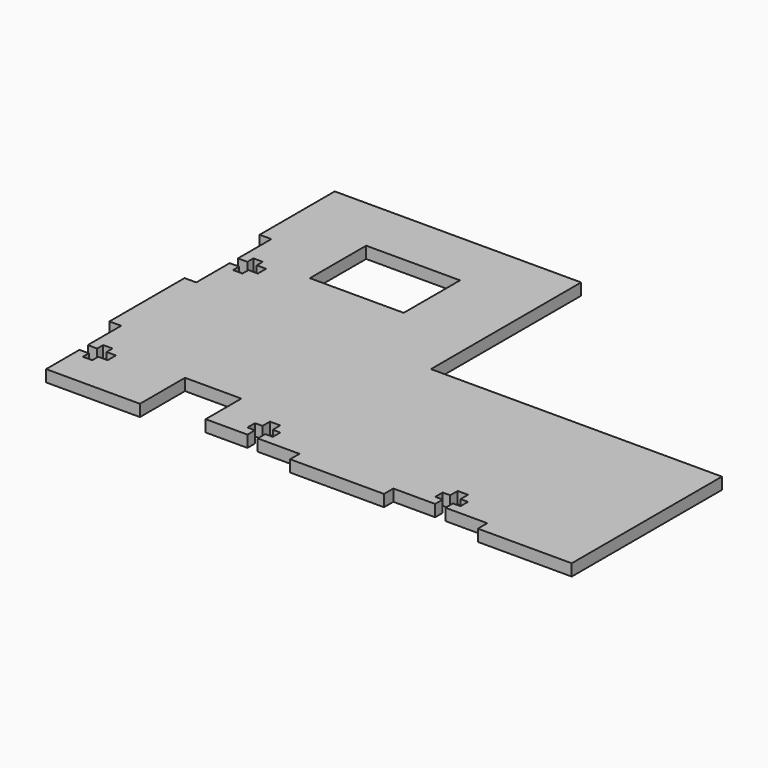
from build123d import *

# Parameters (mm, degrees)
F0_W     = 25.4
F0_H     = 19.05
F1_DEPTH = 3.175


# Not quite as in the source:
# - a feature names something its author has since deleted; it is built from what else it names


with BuildPart() as f1:
    # F0 (on Top) → F1 (new body)
    with BuildSketch(Plane.XY):
        Polygon((2.0699514867, -0.1923768919), (2.0699514867, 50.6076231081), (-61.4300485133, 50.6076231081), (-64.6050485133, 50.6076231081), (-64.6050485133, 25.2076231081), (-61.4300485133, 25.2076231081), (-61.4300485133, 13.9046231081), (-58.8900485133, 13.9046231081), (-58.8900485133, 15.9366231081), (-56.3500485133, 15.9366231081), (-56.3500485133, 13.9046231081), (-53.8100485133, 13.9046231081), (-53.8100485133, 11.1106231081), (-56.3500485133, 11.1106231081), (-56.3500485133, 9.0786231081), (-58.8900485133, 9.0786231081), (-58.8900485133, 11.1106231081), (-61.4300485133, 11.1106231081), (-61.4300485133, -0.1923768919), (-64.6050485133, -0.1923768919), (-64.6050485133, -25.5923768919), (-61.4300485133, -25.5923768919), (-61.4300485133, -36.8953768919), (-58.8900485133, -36.8953768919), (-58.8900485133, -34.8633768919), (-56.3500485133, -34.8633768919), (-56.3500485133, -36.8953768919), (-53.8100485133, -36.8953768919), (-53.8100485133, -39.6893768919), (-56.3500485133, -39.6893768919), (-56.3500485133, -41.7213768919), (-58.8900485133, -41.7213768919), (-58.8900485133, -39.6893768919), (-61.4300485133, -39.6893768919), (-61.4300485133, -50.9923768919), (-36.0300485133, -50.9923768919), (-36.0300485133, -35.7523768919), (-20.7900485133, -35.7523768919), (-20.7900485133, -47.8173768919), (-9.4870485133, -47.8173768919), (-9.4870485133, -45.2773768919), (-11.5190485133, -45.2773768919), (-11.5190485133, -42.7373768919), (-9.4870485133, -42.7373768919), (-9.4870485133, -40.1973768919), (-6.6930485133, -40.1973768919), (-6.6930485133, -42.7373768919), (-4.6610485133, -42.7373768919), (-4.6610485133, -45.2773768919), (-6.6930485133, -45.2773768919), (-6.6930485133, -47.8173768919), (4.6099514867, -47.8173768919), (4.6099514867, -50.9923768919), (30.0099514867, -50.9923768919), (30.0099514867, -47.8173768919), (41.3129514867, -47.8173768919), (41.3129514867, -45.2773768919), (39.2809514867, -45.2773768919), (39.2809514867, -42.7373768919), (41.3129514867, -42.7373768919), (41.3129514867, -40.1973768919), (44.1069514867, -40.1973768919), (44.1069514867, -42.7373768919), (46.1389514867, -42.7373768919), (46.1389514867, -45.2773768919), (44.1069514867, -45.2773768919), (44.1069514867, -47.8173768919), (55.4099514867, -47.8173768919), (55.4099514867, -50.9923768919), (80.8099514867, -50.9923768919), (80.8099514867, -0.1923768919), align=None)
        with Locations((-31.2025573432, 25.8426231081)):
            Rectangle(F0_W, F0_H, mode=Mode.SUBTRACT)
    extrude(amount=F1_DEPTH)


solid = f1.part
